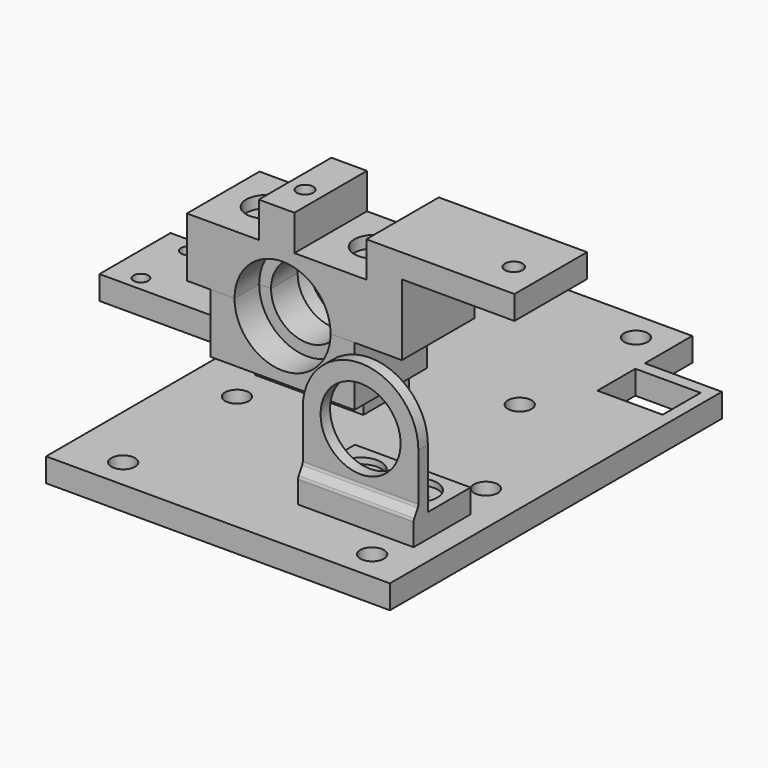
from build123d import *

# Parameters (mm, degrees)
F0_R      = 2
F0_R_2    = 1.5
F0_W      = 27
F0_H      = 15
F0_R_3    = 1.25
F0_W_2    = 2
F0_H_2    = 8
F1_DEPTH  = 4
F4_R      = 1.5
F6_DEPTH  = 4
F7_R      = 1.5
F8_DEPTH  = 10
F9_W      = 6.1
F9_H      = 5.6
F12_DEPTH = 10
F13_R     = 1.4
F14_DEPTH = 6
F15_R     = 1.4
F15_W     = 4
F15_H     = 15.3
F16_DEPTH = 10
F17_W     = 6.1
F17_H     = 5.6
F19_R     = 3.4
F19_R_2   = 1.4
F20_DEPTH = 2
F21_W     = 19.5
F21_H     = 12
F21_R     = 1.5
F22_DEPTH = 4
F23_R     = 3.4
F23_R_2   = 1.5
F24_DEPTH = 1
F25_W     = 19.5
F25_H     = 2
F26_DEPTH = 10
F28_DEPTH = 2
F29_R     = 6.75
F30_DEPTH = 2
F32_DEPTH = 19.5
F33_R     = 1
F34_R     = 1
F35_W     = 15.3
F35_H     = 10
F36_DEPTH = 4
F37_W     = 6
F37_H     = 15.3
F38_DEPTH = 6
F40_W     = 15.3
F40_H     = 4
F41_DEPTH = 19
F42_R     = 1.4
F42_R_2   = 1.5
F43_DEPTH = 20


# Not quite as in the source:
# - a feature of the source that left no trace in its solid (it failed there, or was rolled back) is left out
# - a feature names something its author has since deleted; it is built from what else it names


with BuildPart() as f1:
    # F0 (on Top) → F1 (new body)
    with BuildSketch(Plane.XY):
        Polygon((5, 0), (0, 0), (0, -15), (0, -60), (58, -60), (58, 0), (56, 0), (45, 0), (15, 0), (7, 0), align=None)
        with Locations((9, -55)):
            Circle(F0_R, mode=Mode.SUBTRACT)
        with Locations((9, -31)):
            Circle(F0_R, mode=Mode.SUBTRACT)
        with Locations((11, -20.25)):
            Circle(F0_R_2, mode=Mode.SUBTRACT)
        with Locations((51, -55)):
            Circle(F0_R, mode=Mode.SUBTRACT)
        with Locations((39.5, -43)):
            Circle(F0_R_2, mode=Mode.SUBTRACT)
        with Locations((49, -43)):
            Circle(F0_R_2, mode=Mode.SUBTRACT)
        with Locations((20.5, -31.625)):
            Circle(F0_R_2, mode=Mode.SUBTRACT)
        with Locations((30, -31.625)):
            Circle(F0_R_2, mode=Mode.SUBTRACT)
        with Locations((20.5, -20.25)):
            Circle(F0_R_2, mode=Mode.SUBTRACT)
        with Locations((30, -20.25)):
            Circle(F0_R_2, mode=Mode.SUBTRACT)
        with Locations((39.5, -31.625)):
            Circle(F0_R_2, mode=Mode.SUBTRACT)
        with Locations((51, -31)):
            Circle(F0_R, mode=Mode.SUBTRACT)
        with Locations((39.5, -20.25)):
            Circle(F0_R_2, mode=Mode.SUBTRACT)
        with Locations((49, -20.25)):
            Circle(F0_R_2, mode=Mode.SUBTRACT)
        with Locations((20.5, -9.5)):
            Circle(F0_R, mode=Mode.SUBTRACT)
        with Locations((39.5, -9.5)):
            Circle(F0_R, mode=Mode.SUBTRACT)
        with Locations((-13.5, -7.5)):
            Rectangle(F0_W, F0_H)
        with Locations((-22, -12.5)):
            Circle(F0_R_3, mode=Mode.SUBTRACT)
        with Locations((-22, -2.5)):
            Circle(F0_R_3, mode=Mode.SUBTRACT)
        Polygon((15, 6), (15, 0), (45, 0), (45, 8), (45, 10), (45, 20), (15, 20), (15, 8), align=None)
        with Locations((20.5, 2.75)):
            Circle(F0_R_2, mode=Mode.SUBTRACT)
        with Locations((30, 2.75)):
            Circle(F0_R_2, mode=Mode.SUBTRACT)
        with Locations((20.5, 15)):
            Circle(F0_R, mode=Mode.SUBTRACT)
        with Locations((39.5, 2.75)):
            Circle(F0_R_2, mode=Mode.SUBTRACT)
        with Locations((39.5, 15)):
            Circle(F0_R, mode=Mode.SUBTRACT)
        with Locations((30, -20.25)):
            Circle(F0_R_2)
        with Locations((39.5, -20.25)):
            Circle(F0_R_2)
        with Locations((49, -20.25)):
            Circle(F0_R_2)
        with Locations((30, -31.625)):
            Circle(F0_R_2)
        with Locations((39.5, -31.625)):
            Circle(F0_R_2)
        with Locations((20.5, 2.75)):
            Circle(F0_R_2)
        with Locations((30, 2.75)):
            Circle(F0_R_2)
        with Locations((39.5, 2.75)):
            Circle(F0_R_2)
        with Locations((20.5, -31.625)):
            Circle(F0_R_2)
        Polygon((45, 10), (45, 8), (56, 8), (58, 8), (58, 10), align=None)
        with Locations((57, 4)):
            Rectangle(F0_W_2, F0_H_2)
        Polygon((5, 8), (5, 0), (7, 0), (7, 6), (15, 6), (15, 8), align=None)
    extrude(amount=F1_DEPTH)


with BuildPart() as f6:
    # F4 (on face) → F6 (new body)
    with BuildSketch(Plane.XY.offset(4)):
        Polygon((25.25, -15), (7, -15), (7, -24.6875), (9, -24.6875), (25.25, -24.6875), align=None)
        with Locations((11, -20.25)):
            Circle(F4_R, mode=Mode.SUBTRACT)
        with Locations((20.5, -20.25)):
            Circle(F4_R, mode=Mode.SUBTRACT)
    extrude(amount=F6_DEPTH)

    # F7 (on face) → F8 (join)
    with BuildSketch(Plane.XY.offset(8)):
        Polygon((25.25, -15), (7, -15), (7, -24.6875), (9, -24.6875), (25.25, -24.6875), align=None)
        with Locations((11, -20.25)):
            Circle(F7_R, mode=Mode.SUBTRACT)
        with Locations((20.5, -20.25)):
            Circle(F7_R, mode=Mode.SUBTRACT)
        Polygon((7, -24.6875), (7, -15), (4, -15), (4, -37.3125), (7, -37.3125), align=None)
        with BuildLine():
            Line((9, -24.6875), (7, -24.6875))
            Line((7, -24.6875), (7, -37.3125))
            Line((7, -37.3125), (15.3125, -37.3125))
            Line((15.3125, -37.3125), (15.3125, -31))
            ThreePointArc((15.3125, -31), (13.4636115562, -26.5363884438), (9, -24.6875))
        make_face()
        with BuildLine():
            Line((25.25, -24.6875), (9, -24.6875))
            ThreePointArc((9, -24.6875), (13.4636115562, -26.5363884438), (15.3125, -31))
            Line((15.3125, -31), (15.3125, -37.3125))
            Line((15.3125, -37.3125), (25.25, -37.3125))
            Line((25.25, -37.3125), (25.25, -24.6875))
        make_face()
        Polygon((28.25, -15), (25.25, -15), (25.25, -24.6875), (25.25, -37.3125), (28.25, -37.3125), align=None)
        with Locations((11, -20.25)):
            Circle(F7_R)
        with Locations((20.5, -20.25)):
            Circle(F7_R)
    extrude(amount=F8_DEPTH)

    # F9 (on face) → F10 (revolve, cut)
    with BuildSketch(Plane.XY.offset(18)):
        Polygon((22.225, -25.1), (16.125, -25.1), (16.125, -30.3), (24.225, -30.3), (24.225, -25.1), align=None)
        Polygon((24.225, -15), (16.125, -15), (16.125, -19.5), (22.225, -19.5), (24.225, -19.5), align=None)
        with Locations((19.175, -22.3)):
            Rectangle(F9_W, F9_H)
    revolve(axis=Axis((16.125, -22.3, 18), (0, -1, 0)), mode=Mode.SUBTRACT)

    # F11 (on face) → F12 (cut, through all)
    with BuildSketch(Plane.XY.offset(18)):
        Polygon((8.025, -30.3), (4, -30.3), (4, -37.3125), (28.25, -37.3125), (28.25, -30.3), (24.225, -30.3), align=None)
    extrude(amount=-F12_DEPTH, mode=Mode.SUBTRACT)

    # F13 (on face) → F14 (cut)
    with BuildSketch(Plane.XY.offset(18)):
        with Locations((7.0125, -22.3)):
            Circle(F13_R)
        with Locations((25.2375, -22.3)):
            Circle(F13_R)
    extrude(amount=-F14_DEPTH, mode=Mode.SUBTRACT)

    # F34
    f34_edges = [f6.edges().sort_by_distance(p)[0] for p in [
        (25.25, -19.84375, 8),
        (16.125, -24.6875, 8),
        (7, -19.84375, 8),
    ]]
    fillet(f34_edges, radius=F34_R)


with BuildPart() as f16:
    # F15 (on face) → F16 (new body)
    with BuildSketch(Plane.XY.offset(18)):
        Polygon((25.25, -15), (24.225, -15), (24.225, -19.5), (22.225, -19.5), (22.225, -25.1), (24.225, -25.1), (24.225, -30.3), (28.25, -30.3), (28.25, -15), align=None)
        with Locations((25.2375, -22.3)):
            Circle(F15_R, mode=Mode.SUBTRACT)
        Polygon((7, -15), (4, -15), (4, -30.3), (8.025, -30.3), (8.025, -25.1), (10.025, -25.1), (10.025, -19.5), (8.025, -19.5), (8.025, -15), align=None)
        with Locations((7.0125, -22.3)):
            Circle(F15_R, mode=Mode.SUBTRACT)
        Polygon((24.225, -15), (8.025, -15), (8.025, -19.5), (10.025, -19.5), (10.025, -25.1), (8.025, -25.1), (8.025, -30.3), (24.225, -30.3), (24.225, -25.1), (22.225, -25.1), (22.225, -19.5), (24.225, -19.5), align=None)
        with Locations((2, -22.65)):
            Rectangle(F15_W, F15_H)
        with Locations((30.25, -22.65)):
            Rectangle(F15_W, F15_H)
    extrude(amount=F16_DEPTH)

    # F17 (on face) → F18 (revolve, cut)
    with BuildSketch(Plane(origin=(0, 0, 18), x_dir=(1, 0, 0), z_dir=(0, 0, -1))):
        with Locations((19.175, 22.3)):
            Rectangle(F17_W, F17_H)
        Polygon((24.225, 19.5), (22.225, 19.5), (16.125, 19.5), (16.125, 15), (24.225, 15), align=None)
        Polygon((16.125, 25.1), (22.225, 25.1), (24.225, 25.1), (24.225, 30.3), (16.125, 30.3), align=None)
    revolve(axis=Axis((16.125, -22.3, 18), (0, -1, 0)), mode=Mode.SUBTRACT)

    # F19 (on face) → F20 (cut)
    with BuildSketch(Plane.XY.offset(28)):
        with Locations((7.0125, -22.3)):
            Circle(F19_R)
        with Locations((7.0125, -22.3)):
            Circle(F19_R_2, mode=Mode.SUBTRACT)
        with Locations((25.2375, -22.3)):
            Circle(F19_R)
        with Locations((25.2375, -22.3)):
            Circle(F19_R_2, mode=Mode.SUBTRACT)
    extrude(amount=-F20_DEPTH, mode=Mode.SUBTRACT)

    # F35 (on face) → F36 (join)
    with BuildSketch(Plane.YZ.offset(32.25)):
        with Locations((-22.65, 23)):
            Rectangle(F35_W, F35_H)
    extrude(amount=F36_DEPTH)

    # F37 (on face) → F38 (join)
    with BuildSketch(Plane.XY.offset(28)):
        with Locations((15.125, -22.65)):
            Rectangle(F37_W, F37_H)
        Polygon((32.25, -15), (30.25, -15), (30.25, -30.3), (32.25, -30.3), (36.25, -30.3), (36.25, -15), align=None)
    extrude(amount=F38_DEPTH)

    # F40 (on face) → F41 (join)
    with BuildSketch(Plane.YZ.offset(36.25)):
        with Locations((-22.65, 32)):
            Rectangle(F40_W, F40_H)
    extrude(amount=F41_DEPTH)

    # F42 (on face) → F43 (cut)
    with BuildSketch(Plane.XY.offset(34)):
        with Locations((15.125, -24.3)):
            Circle(F42_R)
        with Locations((50.325, -24.3)):
            Circle(F42_R_2)
    extrude(amount=-F43_DEPTH, mode=Mode.SUBTRACT)


with BuildPart() as f22:
    # F21 (on face) → F22 (new body)
    with BuildSketch(Plane.XY.offset(4)):
        with Locations((44.25, -44)):
            Rectangle(F21_W, F21_H)
        with Locations((39.5, -43)):
            Circle(F21_R, mode=Mode.SUBTRACT)
        with Locations((49, -43)):
            Circle(F21_R, mode=Mode.SUBTRACT)
    extrude(amount=F22_DEPTH)

    # F23 (on face) → F24 (cut)
    with BuildSketch(Plane.XY.offset(8)):
        with Locations((39.5, -43)):
            Circle(F23_R)
        with Locations((39.5, -43)):
            Circle(F23_R_2, mode=Mode.SUBTRACT)
        with Locations((49, -43)):
            Circle(F23_R)
        with Locations((49, -43)):
            Circle(F23_R_2, mode=Mode.SUBTRACT)
    extrude(amount=-F24_DEPTH, mode=Mode.SUBTRACT)

    # F25 (on face) → F26 (join)
    with BuildSketch(Plane.XY.offset(8)):
        with Locations((44.25, -48)):
            Rectangle(F25_W, F25_H)
    extrude(amount=F26_DEPTH)

    # F27 (on face) → F28 (join)
    with BuildSketch(Plane(origin=(0, -47, 0), x_dir=(-1, 0, 0), z_dir=(0, 1, 0))):
        with BuildLine():
            Line((-54, 18), (-34.5, 18))
            ThreePointArc((-34.5, 18), (-44.25, 27.75), (-54, 18))
        make_face()
    extrude(amount=-F28_DEPTH)

    # F29 (on face) → F30 (cut, through all)
    with BuildSketch(Plane(origin=(0, -47, 0), x_dir=(-1, 0, 0), z_dir=(0, 1, 0))):
        with Locations((-44.25, 18)):
            Circle(F29_R)
    extrude(amount=-F30_DEPTH, mode=Mode.SUBTRACT)

    # F31 (on face) → F32 (join)
    with BuildSketch(Plane.YZ.offset(54)):
        Polygon((-49, 9.7320508076), (-50, 8), (-49, 8), align=None)
    extrude(amount=-F32_DEPTH)

    # F33
    f33_edges = [f22.edges().sort_by_distance(p)[0] for p in [
        (44.25, -50, 8),
        (44.25, -49, 9.732051),
    ]]
    fillet(f33_edges, radius=F33_R)


solid = Compound([f1.part, f6.part, f16.part, f22.part])
